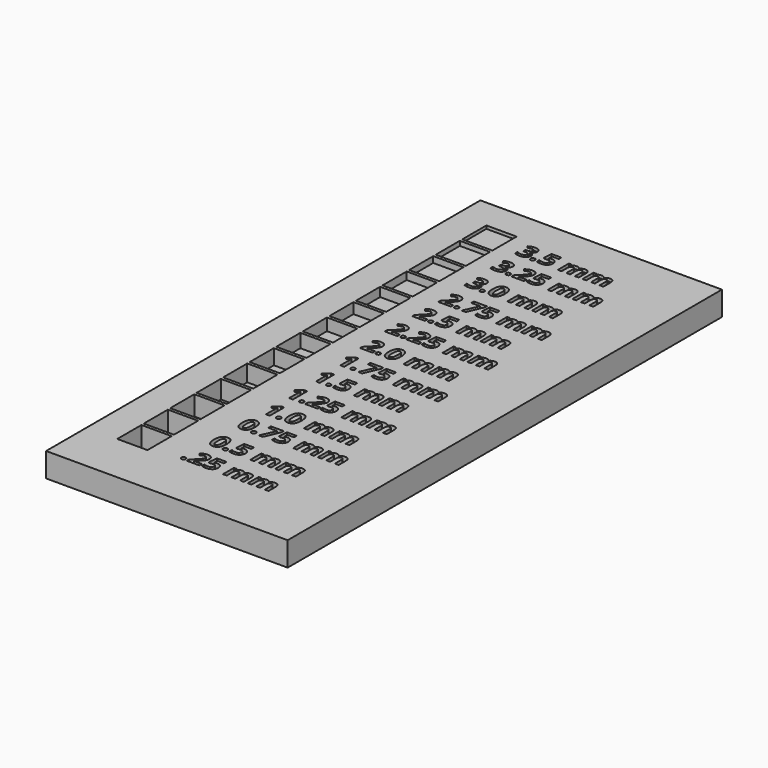
from build123d import *

# Parameters (mm, degrees)
F0_W          = 40
F0_H          = 89.8843802512
F1_DEPTH      = 4
F3_TEXT_SIZE  = 4.1666666667
F4_DEPTH      = 0.5
F2_W          = 5
F2_H          = 5
F5_DEPTH      = 0.5
F6_TEXT_SIZE  = 4.1666666667
F7_DEPTH      = 0.75
F8_DEPTH      = 0.75
F9_TEXT_SIZE  = 4.1666666667
F10_DEPTH     = 1
F11_DEPTH     = 1
F12_TEXT_SIZE = 4.1666666667
F13_DEPTH     = 1.25
F3_W          = 5
F3_H          = 5
F14_DEPTH     = 1.25
F15_TEXT_SIZE = 4.1666666667
F16_DEPTH     = 1.5
F17_DEPTH     = 1.5
F18_TEXT_SIZE = 4.1666666667
F19_DEPTH     = 1.75
F20_DEPTH     = 1.75
F21_TEXT_SIZE = 4.1666666667
F22_DEPTH     = 2
F23_TEXT_SIZE = 4.1666666667
F24_DEPTH     = 2.25
F25_TEXT_SIZE = 4.1666666667
F26_DEPTH     = 2.5
F27_TEXT_SIZE = 4.1666666667
F28_DEPTH     = 2.75
F29_TEXT_SIZE = 4.1666666667
F30_DEPTH     = 3
F31_TEXT_SIZE = 4.1666666667
F32_DEPTH     = 3.25
F33_TEXT_SIZE = 4.1666666667
F34_DEPTH     = 3.5
F35_TEXT_SIZE = 4.1666666667
F36_DEPTH     = 3.75


# Not quite as in the source:
# - Text() gives the source's letters only with a copy of the font that has no kerning and outlines rounded to 1/6400 em; it was checked with that copy


with BuildPart() as f1:
    # F0 (on Top) → F1 (new body)
    with BuildSketch(Plane.XY):
        with Locations((-30, 5.0578098744)):
            Rectangle(F0_W, F0_H)
    extrude(amount=F1_DEPTH)

    # F3 (on face) → F4 (cut)
    with BuildSketch(Plane.XY.offset(4)):
        with Locations((-37.3672095011, 41.0537933827)):
            Text('3.5 mm', F3_TEXT_SIZE, font='Open Sans', font_style=FontStyle.BOLD, text_align=(TextAlign.LEFT, TextAlign.BOTTOM))
    extrude(amount=-F4_DEPTH, mode=Mode.SUBTRACT)

    # F2 (on face) → F5 (cut)
    with BuildSketch(Plane.XY.offset(4)):
        with Locations((-42.5, 42.5)):
            Rectangle(F2_W, F2_H)
    extrude(amount=-F5_DEPTH, mode=Mode.SUBTRACT)

    # F6 (on face) → F7 (cut)
    with BuildSketch(Plane.XY.offset(4)):
        with Locations((-37.269731293, 35.860145703)):
            Text('3.25 mm', F6_TEXT_SIZE, font='Open Sans', font_style=FontStyle.BOLD, text_align=(TextAlign.LEFT, TextAlign.BOTTOM))
    extrude(amount=-F7_DEPTH, mode=Mode.SUBTRACT)

    # F2 (on face) → F8 (cut)
    with BuildSketch(Plane.XY.offset(4)):
        with Locations((-42.5, 37)):
            Rectangle(F2_W, F2_H)
    extrude(amount=-F8_DEPTH, mode=Mode.SUBTRACT)

    # F9 (on face) → F10 (cut)
    with BuildSketch(Plane.XY.offset(4)):
        with Locations((-36.9445017434, 30.064291719)):
            Text('3.0 mm', F9_TEXT_SIZE, font='Open Sans', font_style=FontStyle.BOLD, text_align=(TextAlign.LEFT, TextAlign.BOTTOM))
    extrude(amount=-F10_DEPTH, mode=Mode.SUBTRACT)

    # F2 (on face) → F11 (cut)
    with BuildSketch(Plane.XY.offset(4)):
        with Locations((-42.5, 31.5)):
            Rectangle(F2_W, F2_H)
    extrude(amount=-F11_DEPTH, mode=Mode.SUBTRACT)

    # F12 (on face) → F13 (cut)
    with BuildSketch(Plane.XY.offset(4)):
        with Locations((-36.6318329973, 24.3906318192)):
            Text('2.75 mm', F12_TEXT_SIZE, font='Open Sans', font_style=FontStyle.BOLD, text_align=(TextAlign.LEFT, TextAlign.BOTTOM))
    extrude(amount=-F13_DEPTH, mode=Mode.SUBTRACT)

    # F3 (on face) → F14 (cut)
    with BuildSketch(Plane.XY.offset(4)):
        with Locations((-42.5, 26)):
            Rectangle(F3_W, F3_H)
    extrude(amount=-F14_DEPTH, mode=Mode.SUBTRACT)

    # F15 (on face) → F16 (cut)
    with BuildSketch(Plane.XY.offset(4)):
        with Locations((-36.7654436272, 19.1721934442)):
            Text('2.5 mm', F15_TEXT_SIZE, font='Open Sans', font_style=FontStyle.BOLD, text_align=(TextAlign.LEFT, TextAlign.BOTTOM))
    extrude(amount=-F16_DEPTH, mode=Mode.SUBTRACT)

    # F2 (on face) → F17 (cut)
    with BuildSketch(Plane.XY.offset(4)):
        with Locations((-42.5, 20.5)):
            Rectangle(F2_W, F2_H)
    extrude(amount=-F17_DEPTH, mode=Mode.SUBTRACT)

    # F18 (on face) → F19 (cut)
    with BuildSketch(Plane.XY.offset(4)):
        with Locations((-36.871539435, 13.6055690633)):
            Text('2.25 mm', F18_TEXT_SIZE, font='Open Sans', font_style=FontStyle.BOLD, text_align=(TextAlign.LEFT, TextAlign.BOTTOM))
    extrude(amount=-F19_DEPTH, mode=Mode.SUBTRACT)

    # F2 (on face) → F20 (cut)
    with BuildSketch(Plane.XY.offset(4)):
        with Locations((-42.5, 15)):
            Rectangle(F2_W, F2_H)
    extrude(amount=-F20_DEPTH, mode=Mode.SUBTRACT)

    # F21 (on face) + F2 (on face) → F22 (cut)
    with BuildSketch(Plane.XY.offset(4)):
        with Locations((-36.4727059728, 7.9826633106)):
            Text('2.0 mm', F21_TEXT_SIZE, font='Open Sans', font_style=FontStyle.BOLD, text_align=(TextAlign.LEFT, TextAlign.BOTTOM))
    with BuildSketch(Plane.XY.offset(4)):
        with Locations((-42.5, 9.5)):
            Rectangle(F2_W, F2_H)
    extrude(amount=-F22_DEPTH, mode=Mode.SUBTRACT)

    # F23 (on face) + F2 (on face) → F24 (cut)
    with BuildSketch(Plane.XY.offset(4)):
        with Locations((-36.3493920194, 2.601204239)):
            Text('1.75 mm', F23_TEXT_SIZE, font='Open Sans', font_style=FontStyle.BOLD, text_align=(TextAlign.LEFT, TextAlign.BOTTOM))
    with BuildSketch(Plane.XY.offset(4)):
        with Locations((-42.5, 4)):
            Rectangle(F2_W, F2_H)
    extrude(amount=-F24_DEPTH, mode=Mode.SUBTRACT)

    # F25 (on face) + F2 (on face) → F26 (cut)
    with BuildSketch(Plane.XY.offset(4)):
        with Locations((-36.007390659, -2.8801684062)):
            Text('1.5 mm', F25_TEXT_SIZE, font='Open Sans', font_style=FontStyle.BOLD, text_align=(TextAlign.LEFT, TextAlign.BOTTOM))
    with BuildSketch(Plane.XY.offset(4)):
        with Locations((-42.5, -1.5)):
            Rectangle(F2_W, F2_H)
    extrude(amount=-F26_DEPTH, mode=Mode.SUBTRACT)

    # F27 (on face) + F2 (on face) → F28 (cut)
    with BuildSketch(Plane.XY.offset(4)):
        with Locations((-35.8078034173, -8.6915774001)):
            Text('1.25 mm', F27_TEXT_SIZE, font='Open Sans', font_style=FontStyle.BOLD, text_align=(TextAlign.LEFT, TextAlign.BOTTOM))
    with BuildSketch(Plane.XY.offset(4)):
        with Locations((-42.5, -7)):
            Rectangle(F2_W, F2_H)
    extrude(amount=-F28_DEPTH, mode=Mode.SUBTRACT)

    # F29 (on face) + F2 (on face) → F30 (cut)
    with BuildSketch(Plane.XY.offset(4)):
        with Locations((-35.3007131283, -14.109371636)):
            Text('1.0 mm', F29_TEXT_SIZE, font='Open Sans', font_style=FontStyle.BOLD, text_align=(TextAlign.LEFT, TextAlign.BOTTOM))
    with BuildSketch(Plane.XY.offset(4)):
        with Locations((-42.4799637031, -12.4999635041)):
            Rectangle(F2_W, F2_H)
    extrude(amount=-F30_DEPTH, mode=Mode.SUBTRACT)

    # F31 (on face) + F2 (on face) → F32 (cut)
    with BuildSketch(Plane.XY.offset(4)):
        with Locations((-35.2883845009, -19.3058728518)):
            Text('0.75 mm', F31_TEXT_SIZE, font='Open Sans', font_style=FontStyle.BOLD, text_align=(TextAlign.LEFT, TextAlign.BOTTOM))
    with BuildSketch(Plane.XY.offset(4)):
        with Locations((-42.4599274062, -17.9999270083)):
            Rectangle(F2_W, F2_H)
    extrude(amount=-F32_DEPTH, mode=Mode.SUBTRACT)

    # F33 (on face) + F2 (on face) → F34 (cut)
    with BuildSketch(Plane.XY.offset(4)):
        with Locations((-35.1925062702, -25.3056453034)):
            Text('0.5 mm', F33_TEXT_SIZE, font='Open Sans', font_style=FontStyle.BOLD, text_align=(TextAlign.LEFT, TextAlign.BOTTOM))
    with BuildSketch(Plane.XY.offset(4)):
        with Locations((-42.4398911092, -23.4998905124)):
            Rectangle(F2_W, F2_H)
    extrude(amount=-F34_DEPTH, mode=Mode.SUBTRACT)

    # F35 (on face) + F2 (on face) → F36 (cut)
    with BuildSketch(Plane.XY.offset(4)):
        with Locations((-35.4364910642, -30.6604675258)):
            Text('.25 mm', F35_TEXT_SIZE, font='Open Sans', font_style=FontStyle.BOLD, text_align=(TextAlign.LEFT, TextAlign.BOTTOM))
    with BuildSketch(Plane.XY.offset(4)):
        with Locations((-42.4198548123, -28.9998540165)):
            Rectangle(F2_W, F2_H)
    extrude(amount=-F36_DEPTH, mode=Mode.SUBTRACT)


solid = f1.part
